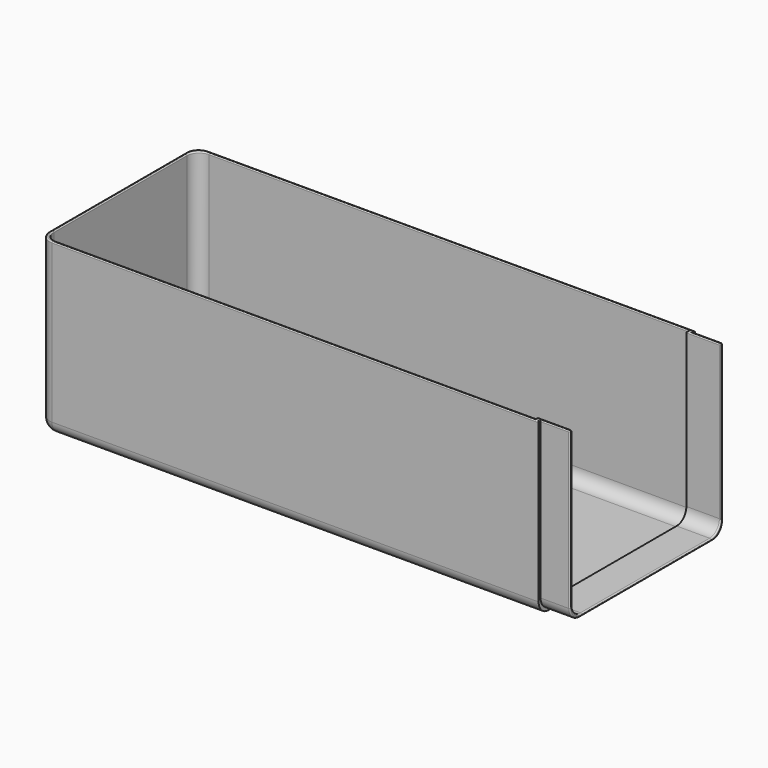
from build123d import *

# Parameters (mm, degrees)
F0_W     = 204
F0_H     = 80
F1_DEPTH = 70
F3_DEPTH = 69
F5_DEPTH = 2
F7_DEPTH = 14
F8_R     = 5
F9_R     = 0.49999


# Not quite as in the source:
# - a fillet or chamfer is up to 0.001 mm smaller than in the source, because OpenCascade refuses the exact size


with BuildPart() as f1:
    # F0 (on Top) → F1 (new body)
    with BuildSketch(Plane.XY):
        Rectangle(F0_W, F0_H)
    extrude(amount=F1_DEPTH)

    # F2 (on face) → F3 (cut)
    with BuildSketch(Plane.XY.offset(70)):
        Polygon((-70.4128742218, 39), (-101, 39), (-101, 20.586034283), (-101, -39), (-57.7337481081, -39), (100, -39), (100, -8.4424866363), (100, 39), align=None)
    extrude(amount=-F3_DEPTH, mode=Mode.SUBTRACT)

    # F4 (on face) → F5 (cut)
    with BuildSketch(Plane.YZ.offset(102)):
        Polygon((38, 2), (38, 70), (-38, 70), (-38, 42.2970801592), (-38, 2), align=None)
    extrude(amount=-F5_DEPTH, mode=Mode.SUBTRACT)

    # F6 (on face) → F7 (join)
    with BuildSketch(Plane(origin=(100, 0, 0), x_dir=(0, -1, 0), z_dir=(-1, 0, 0))):
        Polygon((39, 1), (39, 70), (38, 70), (38, 2), (-38, 2), (-38, 70), (-39, 70), (-39, 1), align=None)
    extrude(amount=-F7_DEPTH)

    # F8
    f8_edges = [f1.edges().sort_by_distance(p)[0] for p in [
        (-0.5, 39, 1),
        (-101, 0, 1),
        (-0.5, -39, 1),
        (0, 40, 0),
        (-102, 0, 0),
        (0, -40, 0),
        (-102, -40, 35),
        (-102, 40, 35),
        (-101, 39, 35.5),
        (-101, -39, 35.5),
        (108, 39, 1),
        (108, -39, 1),
        (107, -38, 2),
        (107, 38, 2),
    ]]
    fillet(f8_edges, radius=F8_R)

    # F9 (radius 0.5 in the source; OpenCascade refuses exactly that, so slightly less here)
    f9_edges = [f1.edges().sort_by_distance(p)[0] for p in [
        (2.5, 40, 70),
        (-100.535534, 38.535534, 70),
        (102, 39.5, 70),
        (-102, 0, 70),
        (108, 39, 70),
        (-100.535534, -38.535534, 70),
        (114, 38.5, 70),
        (2.5, -40, 70),
        (107, 38, 70),
        (102, -39.5, 70),
        (100, 38.5, 70),
        (108, -39, 70),
        (2, 39, 70),
        (114, -38.5, 70),
        (-99.535534, 37.535534, 70),
        (107, -38, 70),
        (-101, 0, 70),
        (100, -38.5, 70),
        (-99.535534, -37.535534, 70),
        (2, -39, 70),
        (114, -39, 38),
        (114, -37.535534, 2.464466),
        (114, 0, 1),
        (114, -38, 38.5),
        (114, 37.535534, 2.464466),
        (114, -36.535534, 3.464466),
        (114, 39, 38),
        (114, 0, 2),
        (114, 36.535534, 3.464466),
        (114, 38, 38.5),
    ]]
    fillet(f9_edges, radius=F9_R)


solid = f1.part
